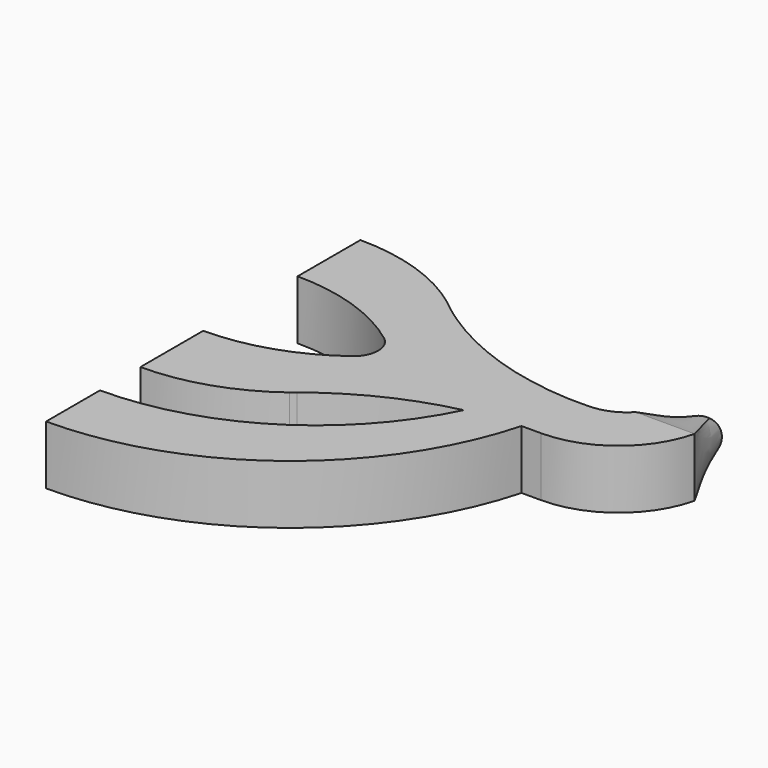
from build123d import *

# Parameters (mm, degrees)
F17_DEPTH = 7.5
F19_DEPTH = 7.5
F20_DEPTH = 7.5


# Not quite as in the source:
# - the arcs of a loft's sections are written as splines that run evenly, so that the points pair up as in the source's solid


with BuildPart() as f9:
    # F2 (on face) → F9 section 0
    with BuildSketch(Plane(origin=(5, -5, 0), x_dir=(0.7071067812, 0.7071067812, 0), z_dir=(0.7071067812, -0.7071067812, 0))):
        with BuildLine():
            add(Edge.make_bspline(
                [(53.6396103068, 0), (53.6396103068, -0.5817764173), (53.7421679492, -1.1634097103), (54.1401264565, -2.2567917229), (54.4354294185, -2.7682714568), (55.1833467639, -3.6596046401), (55.6357771501, -4.0392388103), (56.1396103068, -4.3301270189)],
                knots=[0, 0, 0, 0, 0.3333333333, 0.3333333333, 0.6666666667, 0.6666666667, 1, 1, 1, 1], degree=3))
            add(Edge.make_bspline(
                [(56.1396103068, -4.3301270189), (56.6434434635, -4.6210152276), (57.1984314921, -4.8230143504), (58.3443073448, -5.0250631797), (58.9349132688, -5.0250631797), (60.0807891214, -4.8230143504), (60.6357771501, -4.6210152276), (61.1396103068, -4.3301270189)],
                knots=[0, 0, 0, 0, 0.3333333333, 0.3333333333, 0.6666666667, 0.6666666667, 1, 1, 1, 1], degree=3))
            add(Edge.make_bspline(
                [(61.1396103068, -4.3301270189), (61.6434434635, -4.0392388103), (62.0958738497, -3.6596046401), (62.8437911951, -2.7682714568), (63.1390941571, -2.2567917229), (63.5370526644, -1.1634097103), (63.6396103068, -0.5817764173), (63.6396103068, 0)],
                knots=[0, 0, 0, 0, 0.3333333333, 0.3333333333, 0.6666666667, 0.6666666667, 1, 1, 1, 1], degree=3))
            add(Edge.make_bspline(
                [(63.6396103068, 0), (63.6396103068, 0.5817764173), (63.5370526644, 1.1634097103), (63.1390941571, 2.2567917229), (62.8437911951, 2.7682714568), (62.0958738497, 3.6596046401), (61.6434434635, 4.0392388103), (61.1396103068, 4.3301270189)],
                knots=[0, 0, 0, 0, 0.3333333333, 0.3333333333, 0.6666666667, 0.6666666667, 1, 1, 1, 1], degree=3))
            add(Edge.make_bspline(
                [(61.1396103068, 4.3301270189), (60.6357771501, 4.6210152276), (60.0807891214, 4.8230143504), (58.9349132688, 5.0250631797), (58.3443073448, 5.0250631797), (57.1984314921, 4.8230143504), (56.6434434635, 4.6210152276), (56.1396103068, 4.3301270189)],
                knots=[0, 0, 0, 0, 0.3333333333, 0.3333333333, 0.6666666667, 0.6666666667, 1, 1, 1, 1], degree=3))
            add(Edge.make_bspline(
                [(56.1396103068, 4.3301270189), (55.6357771501, 4.0392388103), (55.1833467639, 3.6596046401), (54.4354294185, 2.7682714568), (54.1401264565, 2.2567917229), (53.7421679492, 1.1634097103), (53.6396103068, 0.5817764173), (53.6396103068, 0)],
                knots=[0, 0, 0, 0, 0.3333333333, 0.3333333333, 0.6666666667, 0.6666666667, 1, 1, 1, 1], degree=3))
        make_face()
    # F8 (on plane+point) → F9 section 1
    with BuildSketch(Plane.XZ.offset(-26.335299015)):
        Polygon((38.9644660941, 7.5), (38.9644660941, 0), (38.9644660941, -7.5), (53.9644660941, -7.5), (53.9644660941, 0), (53.9644660941, 7.5), align=None)
    loft(ruled=True)

    # F16 (on plane+point) → F17 (join, symmetric)
    with BuildSketch(Plane.XY):
        with BuildLine():
            ThreePointArc((38.9644660941, 26.335299015), (34.8752223254, 23.4990929499), (30, 22.5))
            Line((30, 22.5), (30, 7.5))
            ThreePointArc((30, 7.5), (45.2402766064, 12.7723861725), (53.9644660941, 26.335299015))
            Line((53.9644660941, 26.335299015), (38.9644660941, 26.335299015))
        make_face()
    extrude(amount=F17_DEPTH, both=True)

    # F18 (on Top) → F19 (join, symmetric)
    with BuildSketch(Plane.XY):
        Polygon((30, 7.5), (30, 22.5), (25, 22.5), (25, 15), (25, 7.5), align=None)
    extrude(amount=F19_DEPTH, both=True)

    # F18 (on Top) → F20 (join, symmetric)
    with BuildSketch(Plane.XY):
        with BuildLine():
            Line((-50, 40), (-20, 40))
            ThreePointArc((-20, 40), (-34.1886116992, 47.4341649025), (-50, 50))
            Line((-50, 50), (-50, 40))
        make_face()
        with BuildLine():
            Line((25, 15), (25, 22.5))
            ThreePointArc((25, 22.5), (4.5562384252, 26.3545057073), (-14.0947561264, 35.5710670948))
            ThreePointArc((-14.0947561264, 35.5710670948), (-17.1007926042, 37.7143141594), (-20, 40))
            Line((-20, 40), (-50, 40))
            Line((-50, 40), (-50, 30))
            ThreePointArc((-50, 30), (-34.1886116992, 27.4341649025), (-20, 20))
            ThreePointArc((-20, 20), (-18.1598300563, 17.7950849719), (-17.5, 15))
            Line((-17.5, 15), (10, 15))
            Line((10, 15), (25, 15))
        make_face()
        with BuildLine():
            ThreePointArc((-20, -43.971782705), (8.4686762609, -23.4540986425), (25, 7.5))
            ThreePointArc((25, 7.5), (18.3458720417, 6.87456335), (11.7716580953, 5.6711096222))
            ThreePointArc((11.7716580953, 5.6711096222), (-13.5991721952, -22.4348243888), (-50, -32.8560667038))
            Line((-50, -32.8560667038), (-50, -42.8560667038))
            Line((-50, -42.8560667038), (-50, -50))
            ThreePointArc((-50, -50), (-34.7001682709, -48.4780326329), (-20, -43.971782705))
        make_face()
        with BuildLine():
            Line((25, 7.5), (25, 15))
            Line((25, 15), (10, 15))
            Line((10, 15), (11.7716580953, 5.6711096222))
            ThreePointArc((11.7716580953, 5.6711096222), (18.3458720417, 6.87456335), (25, 7.5))
        make_face()
        with BuildLine():
            Line((11.7716580953, 5.6711096222), (10, 15))
            Line((10, 15), (-17.5, 15))
            ThreePointArc((-17.5, 15), (-18.1598300563, 12.2049150281), (-20, 10))
            ThreePointArc((-20, 10), (-34.1886116992, 2.5658350975), (-50, 0))
            Line((-50, 0), (-50, -20))
            ThreePointArc((-50, -20), (-34.1886116992, -17.4341649025), (-20, -10))
            ThreePointArc((-20, -10), (-19.4528820076, -9.5510950315), (-18.9016373284, -9.1072672811))
            ThreePointArc((-18.9016373284, -9.1072672811), (-4.3970359749, 0.0088769739), (11.7716580953, 5.6711096222))
        make_face()
    extrude(amount=F20_DEPTH, both=True)


solid = f9.part
